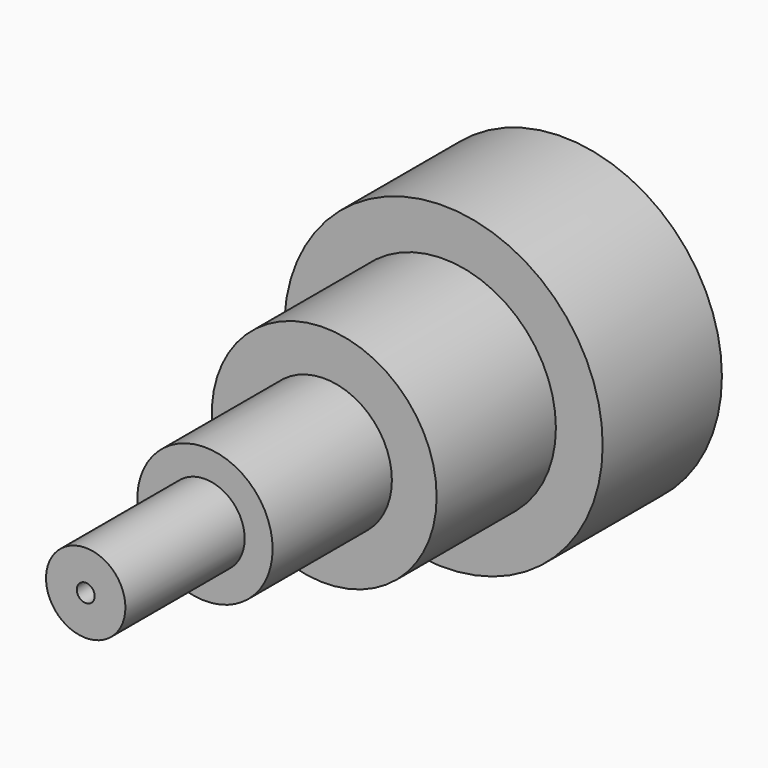
from build123d import *

# Parameters (mm, degrees)
F0_R     = 27.1297247918
F1_DEPTH = 25.4
F2_R     = 19.1590274532
F3_DEPTH = 25.4
F4_R     = 11.5284679065
F5_DEPTH = 25.4
F6_R     = 6.766068174
F6_R_2   = 1.5282390362
F7_DEPTH = 25.4


# Not quite as in the source:
# - the program builds the solid bodies; features that only make, move or delete a surface that nothing else refers to are left out


with BuildPart() as f1:
    # F0 (on Front) → F1 (new body)
    with BuildSketch(Plane.XZ):
        Circle(F0_R)
    extrude(amount=F1_DEPTH)

    # F2 (on face) → F3 (join)
    with BuildSketch(Plane.XZ.offset(25.4)):
        Circle(F2_R)
    extrude(amount=F3_DEPTH)

    # F4 (on face) → F5 (join)
    with BuildSketch(Plane.XZ.offset(50.8)):
        Circle(F4_R)
    extrude(amount=F5_DEPTH)

    # F6 (on face) → F7 (join)
    with BuildSketch(Plane.XZ.offset(76.2)):
        Circle(F6_R)
        Circle(F6_R_2, mode=Mode.SUBTRACT)
    extrude(amount=F7_DEPTH)


solid = f1.part
